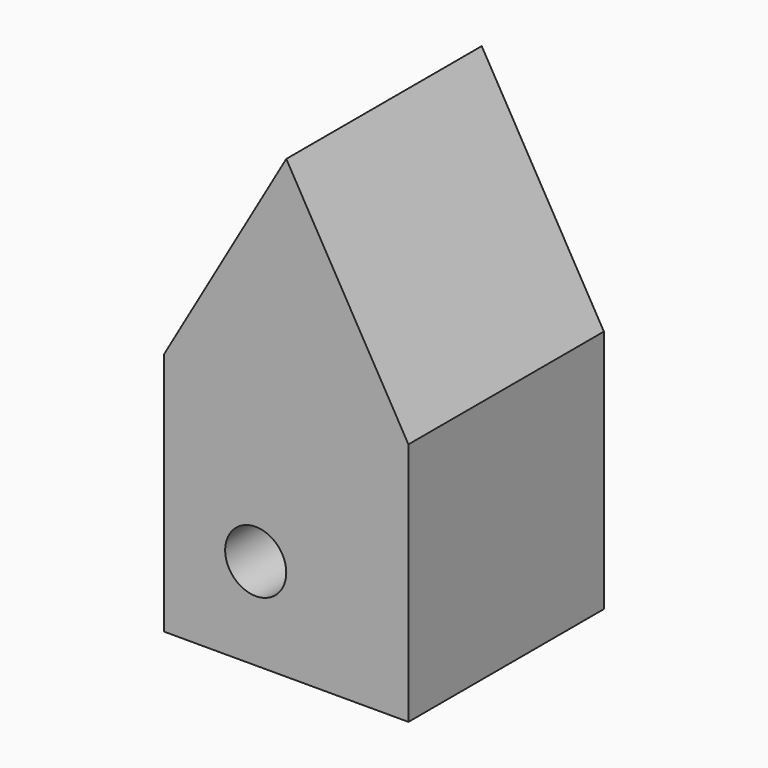
from build123d import *

# Parameters (mm, degrees)
F0_W     = 50.8
F0_H     = 50.8
F0_R     = 6.35
F1_DEPTH = 25.4
F2_DEPTH = 50.8


# Not quite as in the source:
# - a feature names something its author has since deleted; it is built from what else it names


with BuildPart() as f1:
    # F0 (on Front) → F1 (new body)
    with BuildSketch(Plane.XZ):
        Polygon((-25.4, 25.4), (25.4, 25.4), (0, 69.3940905122), align=None)
        Rectangle(F0_W, F0_H)
        with Locations((-6.35, -6.35)):
            Circle(F0_R, mode=Mode.SUBTRACT)
    extrude(amount=F1_DEPTH)

    # F0 (on Front) → F2 (join)
    with BuildSketch(Plane.XZ):
        Rectangle(F0_W, F0_H)
        with Locations((-6.35, -6.35)):
            Circle(F0_R, mode=Mode.SUBTRACT)
        Polygon((-25.4, 25.4), (25.4, 25.4), (0, 69.3940905122), align=None)
    extrude(amount=F2_DEPTH)


solid = f1.part
